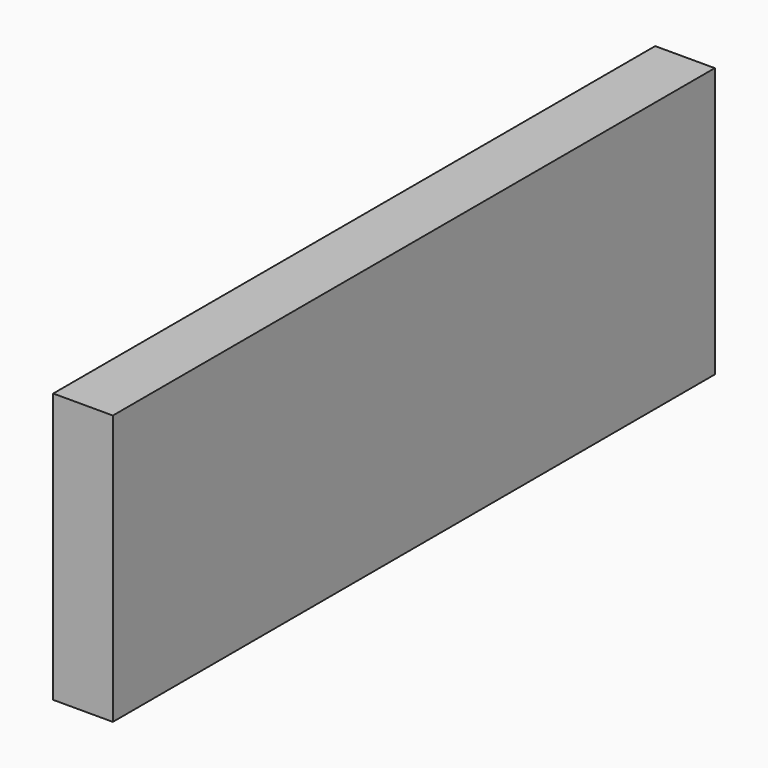
from build123d import *

# Parameters (mm, degrees)
F1_W     = 21
F1_H     = 95
F2_DEPTH = 265


with BuildPart() as f2:
    # F1 (on Front) → F2 (new body)
    with BuildSketch(Plane.XZ):
        with Locations((10.5, 47.5)):
            Rectangle(F1_W, F1_H)
    extrude(amount=F2_DEPTH)


solid = f2.part
